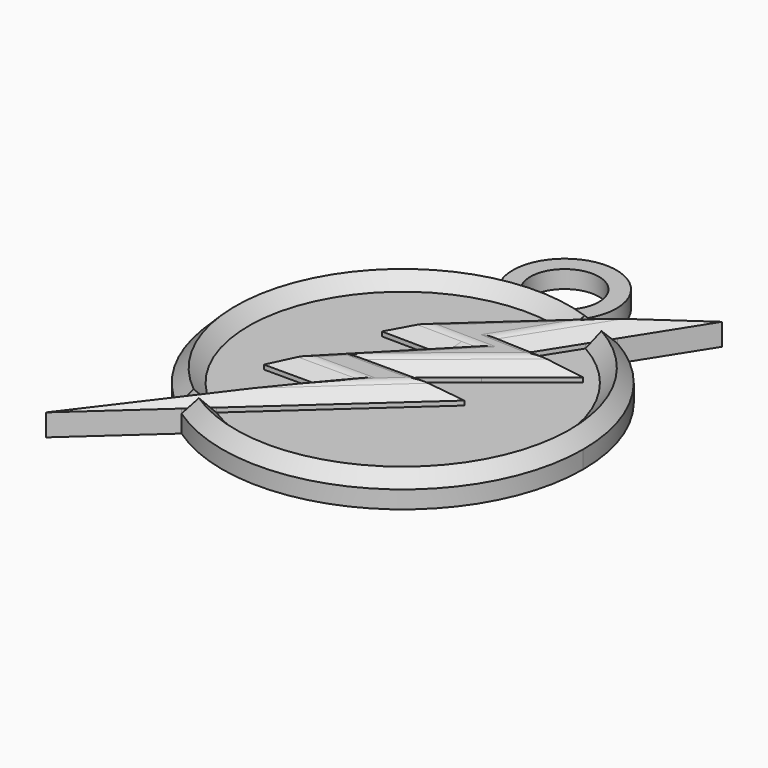
from build123d import *

# Parameters (mm, degrees)
F1_DEPTH      = 4
F2_DEPTH      = 2
F3_DEPTH      = 4
F4_T4_ANGLE   = 191.8794829406
F4_T7_ANGLE   = 191.6152635237
F4_2_T4_ANGLE = 216.7313007881
F4_2_T7_ANGLE = 213.6722162464
F5_T1_DEPTH   = 44.8975853427
F5_T6_DEPTH   = 12.4810064107
F5_T11_DEPTH  = 26.0985725575
F5_T16_DEPTH  = 12.442760274
F5_T21_DEPTH  = 28.0729631379
F5_T23_DEPTH  = 35.0265854945
F5_T28_DEPTH  = 12.5120201061
F5_T30_DEPTH  = 11.8575244819
F5_T35_DEPTH  = 13.9320278094
F5_T40_DEPTH  = 12.6150489639
F5_T45_DEPTH  = 38.8381685856
F6_T1_DEPTH   = 19.5328240955
F6_T3_DEPTH   = 5.6520455224
F6_T5_DEPTH   = 16.5312582393
F6_T7_DEPTH   = 5.740258782
F6_T9_DEPTH   = 5.4658400603
F6_T14_DEPTH  = 14.3536282373
F6_T19_DEPTH  = 7.6900173534
F6_T24_DEPTH  = 3.1100372333
F6_T29_DEPTH  = 12.5427572364
F6_T34_DEPTH  = 18.3278104704
F6_T39_DEPTH  = 9.4173142872
F6_T44_DEPTH  = 3.0038182041
F6_T49_DEPTH  = 11.742181059
F6_T55_DEPTH  = 14.3536282373
F6_T59_DEPTH  = 7.6900173534
F6_T66_DEPTH  = 12.5427572364
F6_T70_DEPTH  = 3.1100372333
F6_T77_DEPTH  = 9.4173142872
F6_T81_DEPTH  = 18.3278104704
F6_T88_DEPTH  = 11.742181059
F6_T92_DEPTH  = 3.0038182041
F7_DEPTH      = 2


# Not quite as in the source:
# - a fillet or chamfer that OpenCascade refuses, or shapes differently, is made with other operations: its cross-section is extruded or revolved along the edge and cut away or added


with BuildPart() as f1:
    # F0 (on Top) → F1 (new body)
    with BuildSketch(Plane.XY):
        with BuildLine():
            ThreePointArc((7.6067055324, 19.0364920861), (6.317476578, 19.5022944723), (5, 19.8808953521))
            ThreePointArc((5, 19.8808953521), (3.9112066982, 20.1234306758), (2.8108329276, 20.3063836823))
            ThreePointArc((2.8108329276, 20.3063836823), (0, 20.5), (-2.8108329276, 20.3063836823))
            ThreePointArc((-2.8108329276, 20.3063836823), (-3.9112066982, 20.1234306758), (-5, 19.8808953521))
            ThreePointArc((-5, 19.8808953521), (-20.0203567241, 4.4085504011), (-12.8882864218, -15.9418340573))
            Line((-12.8882864218, -15.9418340573), (-10.945178398, -13.6547819402))
            ThreePointArc((-10.945178398, -13.6547819402), (-15.4810745708, 8.1600447385), (5.0793558765, 16.7466457501))
            Line((5.0793558765, 16.7466457501), (7.6067055324, 19.0364920861))
        make_face()
    extrude(amount=F1_DEPTH)

    # F0 (on Top) → F2 (join)
    with BuildSketch(Plane.XY):
        with BuildLine():
            Line((-6.9994239003, 5.8029484458), (5.0793558765, 16.7466457501))
            ThreePointArc((5.0793558765, 16.7466457501), (-15.4810745708, 8.1600447385), (-10.945178398, -13.6547819402))
            Line((-10.945178398, -13.6547819402), (-4.1988336978, -5.7142857143))
            Line((-4.1988336978, -5.7142857143), (-11.1988336978, -5.7142857143))
            Line((-11.1988336978, -5.7142857143), (-5.6, 0))
            Line((-5.6, 0), (0, 5.7131427428))
            Line((0, 5.7131427428), (-6.9994239003, 5.8029484458))
        make_face()
    extrude(amount=F2_DEPTH)

    # F4: chamfer of 2 on 2 edges, made by hand


with BuildPart() as f1b:
    # F0 (on Top) → F1, piece 2 (new body)
    with BuildSketch(Plane.XY):
        with BuildLine():
            ThreePointArc((20.5, 0), (17.7262389076, 10.297109021), (10.1555654448, 17.807708738))
            Line((10.1555654448, 17.807708738), (8.5501270855, 15.2690971188))
            ThreePointArc((8.5501270855, 15.2690971188), (15.0976359738, 8.8493721812), (17.5, 0))
            ThreePointArc((17.5, 0), (8.4516512974, -15.3238242729), (-9.336524611, -14.8013279197))
            Line((-9.336524611, -14.8013279197), (-11.6315427767, -16.8806757162))
            ThreePointArc((-11.6315427767, -16.8806757162), (9.5342375961, -18.1479561786), (20.5, 0))
        make_face()
    extrude(amount=F1_DEPTH)

    # F0 (on Top) → F2, piece 2 (join)
    with BuildSketch(Plane.XY):
        with BuildLine():
            ThreePointArc((17.5, 0), (15.0976359738, 8.8493721812), (8.5501270855, 15.2690971188))
            Line((8.5501270855, 15.2690971188), (5.4400217302, 10.3512193653))
            Line((5.4400217302, 10.3512193653), (12.4343353833, 10.0691262568))
            Line((12.4343353833, 10.0691262568), (5.4400217302, 4.4052427373))
            Line((5.4400217302, 4.4052427373), (0, 0))
            Line((0, 0), (7, 0))
            Line((7, 0), (-9.336524611, -14.8013279197))
            ThreePointArc((-9.336524611, -14.8013279197), (8.4516512974, -15.3238242729), (17.5, 0))
        make_face()
    extrude(amount=F2_DEPTH)

    # F4#2: chamfer of 2 on 2 edges, made by hand


with BuildPart() as f3:
    # F0 (on Top) → F3 (new body)
    with BuildSketch(Plane.XY):
        with BuildLine():
            ThreePointArc((-11.6315427767, -16.8806757162), (-12.2688981533, -16.4232803698), (-12.8882864218, -15.9418340573))
            Line((-12.8882864218, -15.9418340573), (-20.5548353552, -24.9654172829))
            Line((-20.5548353552, -24.9654172829), (-11.6315427767, -16.8806757162))
        make_face()
        with BuildLine():
            Line((-10.945178398, -13.6547819402), (-12.8882864218, -15.9418340573))
            ThreePointArc((-12.8882864218, -15.9418340573), (-12.2688981533, -16.4232803698), (-11.6315427767, -16.8806757162))
            Line((-11.6315427767, -16.8806757162), (-9.336524611, -14.8013279197))
            ThreePointArc((-9.336524611, -14.8013279197), (-10.1570424415, -14.2507715174), (-10.945178398, -13.6547819402))
        make_face()
        with BuildLine():
            ThreePointArc((8.5501270855, 15.2690971188), (6.8546691344, 16.1016617483), (5.0793558765, 16.7466457501))
            Line((5.0793558765, 16.7466457501), (-6.9994239003, 5.8029484458))
            Line((-6.9994239003, 5.8029484458), (0, 5.7131427428))
            Line((0, 5.7131427428), (-5.6, 0))
            Line((-5.6, 0), (-11.1988336978, -5.7142857143))
            Line((-11.1988336978, -5.7142857143), (-4.1988336978, -5.7142857143))
            Line((-4.1988336978, -5.7142857143), (-10.945178398, -13.6547819402))
            ThreePointArc((-10.945178398, -13.6547819402), (-10.1570424415, -14.2507715174), (-9.336524611, -14.8013279197))
            Line((-9.336524611, -14.8013279197), (7, 0))
            Line((7, 0), (0, 0))
            Line((0, 0), (5.4400217302, 4.4052427373))
            Line((5.4400217302, 4.4052427373), (12.4343353833, 10.0691262568))
            Line((12.4343353833, 10.0691262568), (5.4400217302, 10.3512193653))
            Line((5.4400217302, 10.3512193653), (8.5501270855, 15.2690971188))
        make_face()
        with BuildLine():
            ThreePointArc((10.1555654448, 17.807708738), (8.9023617482, 18.4661299493), (7.6067055324, 19.0364920861))
            Line((7.6067055324, 19.0364920861), (5.0793558765, 16.7466457501))
            ThreePointArc((5.0793558765, 16.7466457501), (6.8546691344, 16.1016617483), (8.5501270855, 15.2690971188))
            Line((8.5501270855, 15.2690971188), (10.1555654448, 17.807708738))
        make_face()
        with BuildLine():
            Line((15.3954302851, 26.0932848794), (7.6067055324, 19.0364920861))
            ThreePointArc((7.6067055324, 19.0364920861), (8.9023617482, 18.4661299493), (10.1555654448, 17.807708738))
            Line((10.1555654448, 17.807708738), (15.3954302851, 26.0932848794))
        make_face()
    extrude(amount=F3_DEPTH)

    # F5: chamfer of 1.5 on 11 edges, made by hand

    # F5_s2 → F5_t1 (cut)
    with BuildSketch(Plane(origin=(-26.5692425202, -24.0724438327, 0), x_dir=(0, 0, 1), z_dir=(0.7410692771, 0.6714285714, 0))):
        Polygon((2.5, 4.7), (4, 3.2), (4, 4.7), align=None)
    extrude(amount=F5_T1_DEPTH, mode=Mode.SUBTRACT)


with BuildPart() as f4_tool2:
    # F4_s3 → F4_t4 (revolve)
    with BuildSketch(Plane(origin=(0, 0, 0), x_dir=(0, 0, 1), z_dir=(0.9281361418, -0.3722409198, 0))):
        Polygon((2, 17.5), (4, 19.5), (4, 17.5), align=None)
    revolve(axis=Axis((0, 0, 4), (0, 0, -1)), revolution_arc=F4_T4_ANGLE)

    split(bisect_by=Plane.XY.offset(2), keep=Keep.TOP)


with BuildPart() as f1_1:
    add(f1.part)

    # F4_t1: cut F4_tool2
    add(f4_tool2.part, mode=Mode.SUBTRACT)

    # F4_s6 → F4_t7 (revolve, cut)
    with BuildSketch(Plane(origin=(0, 0, 0), x_dir=(0, 0, 1), z_dir=(0.9095275389, -0.4156436646, 0))):
        Polygon((2, 20.5), (4, 18.5), (4, 20.5), align=None)
    revolve(axis=Axis((0, 0, 4), (0, 0, -1)), revolution_arc=F4_T7_ANGLE, mode=Mode.SUBTRACT)

    # F0 (on Top) → F7 (join)
    with BuildSketch(Plane.XY):
        with BuildLine():
            ThreePointArc((2.8108329276, 20.3063836823), (3.9112066982, 20.1234306758), (5, 19.8808953521))
            ThreePointArc((5, 19.8808953521), (0, 28.8931157977), (-5, 19.8808953521))
            ThreePointArc((-5, 19.8808953521), (-3.9112066982, 20.1234306758), (-2.8108329276, 20.3063836823))
            ThreePointArc((-2.8108329276, 20.3063836823), (0, 26.8931157977), (2.8108329276, 20.3063836823))
        make_face()
    extrude(amount=F7_DEPTH)


with BuildPart() as f4_2_tool2:
    # F4_2_s3 → F4_2_t4 (revolve)
    with BuildSketch(Plane(origin=(0, 0, 0), x_dir=(0, 0, 1), z_dir=(-0.6545969301, 0.7559780811, 0))):
        Polygon((2, -17.5), (4, -19.5), (4, -17.5), align=None)
    revolve(axis=Axis((0, 0, 4), (0, 0, 1)), revolution_arc=F4_2_T4_ANGLE)

    split(bisect_by=Plane.XY.offset(2), keep=Keep.TOP)


with BuildPart() as f1b_1:
    add(f1b.part)

    # F4_2_t1: cut F4_2_tool2
    add(f4_2_tool2.part, mode=Mode.SUBTRACT)

    # F4_2_s6 → F4_2_t7 (revolve, cut)
    with BuildSketch(Plane(origin=(0, 0, 0), x_dir=(0, 0, 1), z_dir=(-0.964575687, 0.2638062623, 0))):
        Polygon((2, 20.5), (4, 18.5), (4, 20.5), align=None)
    revolve(axis=Axis((0, 0, 4), (0, 0, -1)), revolution_arc=F4_2_T7_ANGLE, mode=Mode.SUBTRACT)


with BuildPart() as f5_tool4:
    # F5_s5 → F5_t6 (new body)
    with BuildSketch(Plane.YZ.offset(8.6234819288)):
        Polygon((0, 2.5), (-1.5, 4), (0, 4), align=None)
    extrude(amount=-F5_T6_DEPTH)

    split(bisect_by=Plane(origin=(0, 0, 0), x_dir=(0, 0, 1), z_dir=(0.629320391, -0.7771459615, 0)), keep=Keep.TOP)


with BuildPart() as f3_1:
    add(f3.part)

    # F5_t3: cut F5_tool4
    add(f5_tool4.part, mode=Mode.SUBTRACT)


with BuildPart() as f5_tool9:
    # F5_s10 → F5_t11 (new body)
    with BuildSketch(Plane(origin=(15.4321949557, 12.4967450723, 0), x_dir=(0, 0, 1), z_dir=(-0.7771459615, -0.629320391, 0))):
        Polygon((2.5, 0), (4, 1.5), (4, 0), align=None)
    extrude(amount=F5_T11_DEPTH)

    split(bisect_by=Plane(origin=(0, 1.25, 1.25), x_dir=(1, 0, 0), z_dir=(0, 0.7071067812, 0.7071067812)), keep=Keep.TOP)


with BuildPart() as f3_2:
    add(f3_1.part)

    # F5_t8: cut F5_tool9
    add(f5_tool9.part, mode=Mode.SUBTRACT)


with BuildPart() as f5_tool14:
    # F5_s15 → F5_t16 (new body)
    with BuildSketch(Plane(origin=(13.5926436903, -0.5482154936, 0), x_dir=(0, 0, 1), z_dir=(-0.9991876647, 0.0402990155, 0))):
        Polygon((2.5, 10.5620382248), (4, 9.0620382248), (4, 10.5620382248), align=None)
    extrude(amount=F5_T16_DEPTH)

    split(bisect_by=Plane(origin=(-0.7901571012, 0.4997016915, 0), x_dir=(0, 0, 1), z_dir=(0.8451723931, -0.5344938035, 0)), keep=Keep.TOP)


with BuildPart() as f3_3:
    add(f3_2.part)

    # F5_t13: cut F5_tool14
    add(f5_tool14.part, mode=Mode.SUBTRACT)


with BuildPart() as f5_tool19:
    # F5_s20 → F5_t21 (new body)
    with BuildSketch(Plane(origin=(18.247410319, 28.8538563855, 0), x_dir=(0, 0, 1), z_dir=(-0.5344938035, -0.8451723931, 0))):
        Polygon((2.5, 0.9349064259), (4, 2.4349064259), (4, 0.9349064259), align=None)
    extrude(amount=F5_T21_DEPTH)

    split(bisect_by=Plane(origin=(0.2631936405, 6.5257137352, 6.5310191124), x_dir=(-0.9991876647, 0.0402990155, 0), z_dir=(0.0284957071, 0.7065323734, 0.7071067812)), keep=Keep.TOP)


with BuildPart() as f3_4:
    add(f3_3.part)

    # F5_t18: cut F5_tool19
    add(f5_tool19.part, mode=Mode.SUBTRACT)

    # F5_s24 → F5_t23 (cut)
    with BuildSketch(Plane(origin=(22.1418667552, 20.0611230603, 0), x_dir=(0, 0, 1), z_dir=(-0.7410692771, -0.6714285714, 0))):
        Polygon((2.5, 9), (4, 7.5), (4, 9), align=None)
    extrude(amount=F5_T23_DEPTH, mode=Mode.SUBTRACT)


with BuildPart() as f5_tool26:
    # F5_s27 → F5_t28 (new body)
    with BuildSketch(Plane(origin=(-8.7270734415, 0.1119722104, 0), x_dir=(0, 0, 1), z_dir=(0.9999177, -0.0128293861, 0))):
        Polygon((2.5, -5.7126725514), (4, -7.2126725514), (4, -5.7126725514), align=None)
    extrude(amount=F5_T28_DEPTH)

    split(bisect_by=Plane(origin=(-2.856, 2.799439944, 0), x_dir=(0, 0, 1), z_dir=(-0.7141428429, 0.7, 0)), keep=Keep.TOP)


with BuildPart() as f3_5:
    add(f3_4.part)

    # F5_t25: cut F5_tool26
    add(f5_tool26.part, mode=Mode.SUBTRACT)

    # F5_s31 → F5_t30 (cut)
    with BuildSketch(Plane(origin=(-2.7428571429, -2.7994168489, 0), x_dir=(0, 0, 1), z_dir=(-0.6998542122, -0.7142857143, 0))):
        Polygon((2.5, 4), (4, 2.5), (4, 4), align=None)
    extrude(amount=F5_T30_DEPTH, mode=Mode.SUBTRACT)


with BuildPart() as f5_tool33:
    # F5_s34 → F5_t35 (new body)
    with BuildSketch(Plane(origin=(-2.744, -2.799439944, 0), x_dir=(0, 0, 1), z_dir=(0.7, 0.7141428429, 0))):
        Polygon((2.5, -3.99919992), (4, -2.49919992), (4, -3.99919992), align=None)
    extrude(amount=F5_T35_DEPTH)

    split(bisect_by=Plane(origin=(0.0206083084, 1.6062040743, -1.6063362757), x_dir=(0.9999177, -0.0128293861, 0), z_dir=(-0.0090717459, -0.7070485863, 0.7071067812)), keep=Keep.TOP)


with BuildPart() as f3_6:
    add(f3_5.part)

    # F5_t32: cut F5_tool33
    add(f5_tool33.part, mode=Mode.SUBTRACT)


with BuildPart() as f5_tool38:
    # F5_s39 → F5_t40 (new body)
    with BuildSketch(Plane.YZ.offset(-12.9563581797)):
        Polygon((-5.7142857143, 2.5), (-4.2142857143, 4), (-5.7142857143, 4), align=None)
    extrude(amount=F5_T40_DEPTH)

    split(bisect_by=Plane(origin=(0.3810425154, -0.3237384769, 0), x_dir=(0, 0, 1), z_dir=(-0.7620850308, 0.6474769539, 0)), keep=Keep.TOP)


with BuildPart() as f3_7:
    add(f3_6.part)

    # F5_t37: cut F5_tool38
    add(f5_tool38.part, mode=Mode.SUBTRACT)


with BuildPart() as f5_tool43:
    # F5_s44 → F5_t45 (new body)
    with BuildSketch(Plane(origin=(-25.9546183807, -30.5487724767, 0), x_dir=(0, 0, 1), z_dir=(0.6474769539, 0.7620850308, 0))):
        Polygon((2.5, 0.5), (4, 2), (4, 0.5), align=None)
    extrude(amount=F5_T45_DEPTH)

    split(bisect_by=Plane(origin=(0, -4.1071428571, 4.1071428571), x_dir=(1, 0, 0), z_dir=(0, -0.7071067812, 0.7071067812)), keep=Keep.TOP)


with BuildPart() as f3_8:
    add(f3_7.part)

    # F5_t42: cut F5_tool43
    add(f5_tool43.part, mode=Mode.SUBTRACT)

    # F6: fillet of radius 1 on 13 edges, made by hand

    # F6_s2 → F6_t1 (cut)
    with BuildSketch(Plane(origin=(15.5795084063, 14.1154510057, 0), x_dir=(0, 0, 1), z_dir=(-0.7410692771, -0.6714285714, 0))):
        with BuildLine():
            ThreePointArc((4, 7.0857864376), (3.9238795325, 7.46846987), (3.7071067812, 7.7928932188))
            Line((3.7071067812, 7.7928932188), (4, 7.5))
            Line((4, 7.5), (4, 7.0857864376))
        make_face()
    extrude(amount=F6_T1_DEPTH, mode=Mode.SUBTRACT)

    # F6_s4 → F6_t3 (cut)
    with BuildSketch(Plane(origin=(-4.2919621914, 0.0550677723, 0), x_dir=(0, 0, 1), z_dir=(0.9999177, -0.0128293861, 0))):
        with BuildLine():
            ThreePointArc((4, -7.6268861138), (3.9238795325, -7.2442026814), (3.7071067812, -6.9197793326))
            Line((3.7071067812, -6.9197793326), (4, -7.2126725514))
            Line((4, -7.2126725514), (4, -7.6268861138))
        make_face()
    extrude(amount=F6_T3_DEPTH, mode=Mode.SUBTRACT)

    # F6_s6 → F6_t5 (cut)
    with BuildSketch(Plane(origin=(-10.5215995116, -9.5328503656, 0), x_dir=(0, 0, 1), z_dir=(0.7410692771, 0.6714285714, 0))):
        with BuildLine():
            ThreePointArc((3.7071067812, 3.4928932188), (3.9238795325, 3.16846987), (4, 2.7857864376))
            Line((4, 2.7857864376), (4, 3.2))
            Line((4, 3.2), (3.7071067812, 3.4928932188))
        make_face()
    extrude(amount=F6_T5_DEPTH, mode=Mode.SUBTRACT)

    # F6_s8 → F6_t7 (cut)
    with BuildSketch(Plane.YZ.offset(-8.6646737581)):
        with BuildLine():
            ThreePointArc((-3.8000721519, 4), (-4.1827555843, 3.9238795325), (-4.5071789331, 3.7071067812))
            Line((-4.5071789331, 3.7071067812), (-4.2142857143, 4))
            Line((-4.2142857143, 4), (-3.8000721519, 4))
        make_face()
    extrude(amount=F6_T7_DEPTH, mode=Mode.SUBTRACT)

    # F6_s10 → F6_t9 (cut)
    with BuildSketch(Plane(origin=(-2.7428571429, -2.7994168489, 0), x_dir=(0, 0, 1), z_dir=(-0.6998542122, -0.7142857143, 0))):
        with BuildLine():
            ThreePointArc((4, 2.0857864376), (3.9238795325, 2.46846987), (3.7071067812, 2.7928932188))
            Line((3.7071067812, 2.7928932188), (4, 2.5))
            Line((4, 2.5), (4, 2.0857864376))
        make_face()
    extrude(amount=F6_T9_DEPTH, mode=Mode.SUBTRACT)


with BuildPart() as f6_tool12:
    # F6_s13 → F6_t14 (new body)
    with BuildSketch(Plane(origin=(11.9599620904, 18.9117810419, 0), x_dir=(0, 0, 1), z_dir=(-0.5344938035, -0.8451723931, 0))):
        with BuildLine():
            ThreePointArc((4, 2.8491199883), (3.9238795325, 2.4664365559), (3.7071067812, 2.1420132071))
            Line((3.7071067812, 2.1420132071), (4, 2.4349064259))
            Line((4, 2.4349064259), (4, 2.8491199883))
        make_face()
    extrude(amount=F6_T14_DEPTH)

    split(bisect_by=Plane(origin=(0.2631936405, 6.5257137352, 6.5310191124), x_dir=(-0.9991876647, 0.0402990155, 0), z_dir=(0.0284957071, 0.7065323734, 0.7071067812)), keep=Keep.TOP)


with BuildPart() as f3_9:
    add(f3_8.part)

    # F6_t11: cut F6_tool12
    add(f6_tool12.part, mode=Mode.SUBTRACT)


with BuildPart() as f6_tool17:
    # F6_s18 → F6_t19 (new body)
    with BuildSketch(Plane(origin=(9.0674940614, -0.3657081614, 0), x_dir=(0, 0, 1), z_dir=(-0.9991876647, 0.0402990155, 0))):
        with BuildLine():
            ThreePointArc((4, 8.6478246624), (3.9238795325, 9.0305080948), (3.7071067812, 9.3549314436))
            Line((3.7071067812, 9.3549314436), (4, 9.0620382248))
            Line((4, 9.0620382248), (4, 8.6478246624))
        make_face()
    extrude(amount=F6_T19_DEPTH)

    split(bisect_by=Plane(origin=(0.6613869407, -0.4182664087, 0.7825467871), x_dir=(0.5344938035, 0.8451723931, 0), z_dir=(0.5976271304, -0.377944193, 0.7071067812)), keep=Keep.TOP)


with BuildPart() as f3_10:
    add(f3_9.part)

    # F6_t16: cut F6_tool17
    add(f6_tool17.part, mode=Mode.SUBTRACT)


with BuildPart() as f6_tool22:
    # F6_s23 → F6_t24 (new body)
    with BuildSketch(Plane(origin=(1.3596181679, -0.0174445022, 0), x_dir=(0, 0, 1), z_dir=(0.9999177, -0.0128293861, 0))):
        with BuildLine():
            ThreePointArc((4, -7.6268861138), (3.9238795325, -7.2442026814), (3.7071067812, -6.9197793326))
            Line((3.7071067812, -6.9197793326), (4, -7.2126725514))
            Line((4, -7.2126725514), (4, -7.6268861138))
        make_face()
    extrude(amount=F6_T24_DEPTH)

    split(bisect_by=Plane(origin=(-2.3206785536, 2.274719972, 3.24959996), x_dir=(-0.7, -0.7141428429, 0), z_dir=(-0.5049752469, 0.4949747468, 0.7071067812)), keep=Keep.TOP)


with BuildPart() as f3_11:
    add(f3_10.part)

    # F6_t21: cut F6_tool22
    add(f6_tool22.part, mode=Mode.SUBTRACT)


with BuildPart() as f6_tool27:
    # F6_s28 → F6_t29 (new body)
    with BuildSketch(Plane(origin=(-2.7437856705, -2.7992212842, 0), x_dir=(0, 0, 1), z_dir=(0.7, 0.7141428429, 0))):
        with BuildLine():
            ThreePointArc((4, -2.0849863576), (3.9238795325, -2.46766979), (3.7071067812, -2.7920931388))
            Line((3.7071067812, -2.7920931388), (4, -2.49919992))
            Line((4, -2.49919992), (4, -2.0849863576))
        make_face()
    extrude(amount=F6_T29_DEPTH)

    split(bisect_by=Plane(origin=(0.0206083084, 1.6062040743, -1.6063362757), x_dir=(0.9999177, -0.0128293861, 0), z_dir=(-0.0090717459, -0.7070485863, 0.7071067812)), keep=Keep.TOP)


with BuildPart() as f3_12:
    add(f3_11.part)

    # F6_t26: cut F6_tool27
    add(f6_tool27.part, mode=Mode.SUBTRACT)


with BuildPart() as f6_tool32:
    # F6_s33 → F6_t34 (new body)
    with BuildSketch(Plane(origin=(10.1467341546, 8.2166633075, 0), x_dir=(0, 0, 1), z_dir=(-0.7771459615, -0.629320391, 0))):
        with BuildLine():
            ThreePointArc((4, 1.9142135624), (3.9238795325, 1.53153013), (3.7071067812, 1.2071067812))
            Line((3.7071067812, 1.2071067812), (4, 1.5))
            Line((4, 1.5), (4, 1.9142135624))
        make_face()
    extrude(amount=F6_T34_DEPTH)

    split(bisect_by=Plane(origin=(0, 1.25, 1.25), x_dir=(1, 0, 0), z_dir=(0, 0.7071067812, 0.7071067812)), keep=Keep.TOP)


with BuildPart() as f3_13:
    add(f3_12.part)

    # F6_t31: cut F6_tool32
    add(f6_tool32.part, mode=Mode.SUBTRACT)


with BuildPart() as f6_tool37:
    # F6_s38 → F6_t39 (new body)
    with BuildSketch(Plane.YZ.offset(-5.2714032343)):
        with BuildLine():
            ThreePointArc((-1.2071067812, 3.7071067812), (-1.53153013, 3.9238795325), (-1.9142135624, 4))
            Line((-1.9142135624, 4), (-1.5, 4))
            Line((-1.5, 4), (-1.2071067812, 3.7071067812))
        make_face()
    extrude(amount=F6_T39_DEPTH)

    split(bisect_by=Plane(origin=(0.7866504888, -0.9714324518, 1.25), x_dir=(0.7771459615, 0.629320391, 0), z_dir=(0.4449967161, -0.5495251793, 0.7071067812)), keep=Keep.TOP)


with BuildPart() as f3_14:
    add(f3_13.part)

    # F6_t36: cut F6_tool37
    add(f6_tool37.part, mode=Mode.SUBTRACT)


with BuildPart() as f6_tool42:
    # F6_s43 → F6_t44 (new body)
    with BuildSketch(Plane.YZ.offset(-2.924414976)):
        with BuildLine():
            ThreePointArc((-3.8000721519, 4), (-4.1827555843, 3.9238795325), (-4.5071789331, 3.7071067812))
            Line((-4.5071789331, 3.7071067812), (-4.2142857143, 4))
            Line((-4.2142857143, 4), (-3.8000721519, 4))
        make_face()
    extrude(amount=F6_T44_DEPTH)

    split(bisect_by=Plane(origin=(-0.7620850308, 0.6474769539, 1), x_dir=(-0.6474769539, -0.7620850308, 0), z_dir=(-0.5388754931, 0.4578353448, 0.7071067812)), keep=Keep.TOP)


with BuildPart() as f3_15:
    add(f3_14.part)

    # F6_t41: cut F6_tool42
    add(f6_tool42.part, mode=Mode.SUBTRACT)


with BuildPart() as f6_tool47:
    # F6_s48 → F6_t49 (new body)
    with BuildSketch(Plane(origin=(-9.4126080245, -11.078707332, 0), x_dir=(0, 0, 1), z_dir=(0.6474769539, 0.7620850308, 0))):
        with BuildLine():
            ThreePointArc((4, 2.4142135624), (3.9238795325, 2.03153013), (3.7071067812, 1.7071067812))
            Line((3.7071067812, 1.7071067812), (4, 2))
            Line((4, 2), (4, 2.4142135624))
        make_face()
    extrude(amount=F6_T49_DEPTH)

    split(bisect_by=Plane(origin=(0, -4.1071428571, 4.1071428571), x_dir=(1, 0, 0), z_dir=(0, -0.7071067812, 0.7071067812)), keep=Keep.TOP)


with BuildPart() as f3_16:
    add(f3_15.part)

    # F6_t46: cut F6_tool47
    add(f6_tool47.part, mode=Mode.SUBTRACT)


with BuildPart() as f6_tool53:
    # F6_s54 → F6_t55 (new body)
    with BuildSketch(Plane(origin=(11.9599620904, 18.9117810419, 0), x_dir=(0, 0, 1), z_dir=(-0.5344938035, -0.8451723931, 0))):
        with BuildLine():
            ThreePointArc((4, 2.8491199883), (3.9238795325, 2.4664365559), (3.7071067812, 2.1420132071))
            Line((3.7071067812, 2.1420132071), (4, 2.4349064259))
            Line((4, 2.4349064259), (4, 2.8491199883))
        make_face()
    extrude(amount=F6_T55_DEPTH)

    split(bisect_by=Plane(origin=(0.2631936405, 6.5257137352, 6.5310191124), x_dir=(0.9991876647, -0.0402990155, 0), z_dir=(-0.0284957071, -0.7065323734, -0.7071067812)), keep=Keep.TOP)


with BuildPart() as f6_tool57:
    # F6_s58 → F6_t59 (new body)
    with BuildSketch(Plane(origin=(9.0674940614, -0.3657081614, 0), x_dir=(0, 0, 1), z_dir=(-0.9991876647, 0.0402990155, 0))):
        with BuildLine():
            ThreePointArc((4, 8.6478246624), (3.9238795325, 9.0305080948), (3.7071067812, 9.3549314436))
            Line((3.7071067812, 9.3549314436), (4, 9.0620382248))
            Line((4, 9.0620382248), (4, 8.6478246624))
        make_face()
    extrude(amount=F6_T59_DEPTH)

    split(bisect_by=Plane(origin=(0.6613869407, -0.4182664087, 0.7825467871), x_dir=(-0.5344938035, -0.8451723931, 0), z_dir=(-0.5976271304, 0.377944193, -0.7071067812)), keep=Keep.TOP)


with BuildPart() as f6_tool53_1:
    add(f6_tool53.part)

    # F6_t61: intersect F6_tool57
    add(f6_tool57.part, mode=Mode.INTERSECT)


with BuildPart() as f3_17:
    add(f3_16.part)

    # F6_t51: cut F6_tool53
    add(f6_tool53_1.part, mode=Mode.SUBTRACT)


with BuildPart() as f6_tool64:
    # F6_s65 → F6_t66 (new body)
    with BuildSketch(Plane(origin=(-2.7437856705, -2.7992212842, 0), x_dir=(0, 0, 1), z_dir=(0.7, 0.7141428429, 0))):
        with BuildLine():
            ThreePointArc((4, -2.0849863576), (3.9238795325, -2.46766979), (3.7071067812, -2.7920931388))
            Line((3.7071067812, -2.7920931388), (4, -2.49919992))
            Line((4, -2.49919992), (4, -2.0849863576))
        make_face()
    extrude(amount=F6_T66_DEPTH)

    split(bisect_by=Plane(origin=(0.0206083084, 1.6062040743, -1.6063362757), x_dir=(-0.9999177, 0.0128293861, 0), z_dir=(0.0090717459, 0.7070485863, -0.7071067812)), keep=Keep.TOP)


with BuildPart() as f6_tool68:
    # F6_s69 → F6_t70 (new body)
    with BuildSketch(Plane(origin=(1.3596181679, -0.0174445022, 0), x_dir=(0, 0, 1), z_dir=(0.9999177, -0.0128293861, 0))):
        with BuildLine():
            ThreePointArc((4, -7.6268861138), (3.9238795325, -7.2442026814), (3.7071067812, -6.9197793326))
            Line((3.7071067812, -6.9197793326), (4, -7.2126725514))
            Line((4, -7.2126725514), (4, -7.6268861138))
        make_face()
    extrude(amount=F6_T70_DEPTH)

    split(bisect_by=Plane(origin=(-2.3206785536, 2.274719972, 3.24959996), x_dir=(0.7, 0.7141428429, 0), z_dir=(0.5049752469, -0.4949747468, -0.7071067812)), keep=Keep.TOP)


with BuildPart() as f6_tool64_1:
    add(f6_tool64.part)

    # F6_t72: intersect F6_tool68
    add(f6_tool68.part, mode=Mode.INTERSECT)


with BuildPart() as f3_18:
    add(f3_17.part)

    # F6_t62: cut F6_tool64
    add(f6_tool64_1.part, mode=Mode.SUBTRACT)


with BuildPart() as f6_tool75:
    # F6_s76 → F6_t77 (new body)
    with BuildSketch(Plane.YZ.offset(-5.2714032343)):
        with BuildLine():
            ThreePointArc((-1.2071067812, 3.7071067812), (-1.53153013, 3.9238795325), (-1.9142135624, 4))
            Line((-1.9142135624, 4), (-1.5, 4))
            Line((-1.5, 4), (-1.2071067812, 3.7071067812))
        make_face()
    extrude(amount=F6_T77_DEPTH)

    split(bisect_by=Plane(origin=(0.7866504888, -0.9714324518, 1.25), x_dir=(-0.7771459615, -0.629320391, 0), z_dir=(-0.4449967161, 0.5495251793, -0.7071067812)), keep=Keep.TOP)


with BuildPart() as f6_tool79:
    # F6_s80 → F6_t81 (new body)
    with BuildSketch(Plane(origin=(10.1467341546, 8.2166633075, 0), x_dir=(0, 0, 1), z_dir=(-0.7771459615, -0.629320391, 0))):
        with BuildLine():
            ThreePointArc((4, 1.9142135624), (3.9238795325, 1.53153013), (3.7071067812, 1.2071067812))
            Line((3.7071067812, 1.2071067812), (4, 1.5))
            Line((4, 1.5), (4, 1.9142135624))
        make_face()
    extrude(amount=F6_T81_DEPTH)

    split(bisect_by=Plane(origin=(0, 1.25, 1.25), x_dir=(1, 0, 0), z_dir=(0, -0.7071067812, -0.7071067812)), keep=Keep.TOP)


with BuildPart() as f6_tool75_1:
    add(f6_tool75.part)

    # F6_t83: intersect F6_tool79
    add(f6_tool79.part, mode=Mode.INTERSECT)


with BuildPart() as f3_19:
    add(f3_18.part)

    # F6_t73: cut F6_tool75
    add(f6_tool75_1.part, mode=Mode.SUBTRACT)


with BuildPart() as f6_tool86:
    # F6_s87 → F6_t88 (new body)
    with BuildSketch(Plane(origin=(-9.4126080245, -11.078707332, 0), x_dir=(0, 0, 1), z_dir=(0.6474769539, 0.7620850308, 0))):
        with BuildLine():
            ThreePointArc((4, 2.4142135624), (3.9238795325, 2.03153013), (3.7071067812, 1.7071067812))
            Line((3.7071067812, 1.7071067812), (4, 2))
            Line((4, 2), (4, 2.4142135624))
        make_face()
    extrude(amount=F6_T88_DEPTH)

    split(bisect_by=Plane(origin=(0, -4.1071428572, 4.1071428572), x_dir=(1, 0, 0), z_dir=(0, 0.7071067812, -0.7071067812)), keep=Keep.TOP)


with BuildPart() as f6_tool90:
    # F6_s91 → F6_t92 (new body)
    with BuildSketch(Plane.YZ.offset(-2.924414976)):
        with BuildLine():
            ThreePointArc((-3.8000721519, 4), (-4.1827555843, 3.9238795325), (-4.5071789331, 3.7071067812))
            Line((-4.5071789331, 3.7071067812), (-4.2142857143, 4))
            Line((-4.2142857143, 4), (-3.8000721519, 4))
        make_face()
    extrude(amount=F6_T92_DEPTH)

    split(bisect_by=Plane(origin=(-0.7620850308, 0.6474769539, 1), x_dir=(0.6474769539, 0.7620850308, 0), z_dir=(0.5388754931, -0.4578353448, -0.7071067812)), keep=Keep.TOP)


with BuildPart() as f6_tool86_1:
    add(f6_tool86.part)

    # F6_t94: intersect F6_tool90
    add(f6_tool90.part, mode=Mode.INTERSECT)


with BuildPart() as f3_20:
    add(f3_19.part)

    # F6_t84: cut F6_tool86
    add(f6_tool86_1.part, mode=Mode.SUBTRACT)


solid = Compound([f1_1.part, f1b_1.part, f3_20.part])
